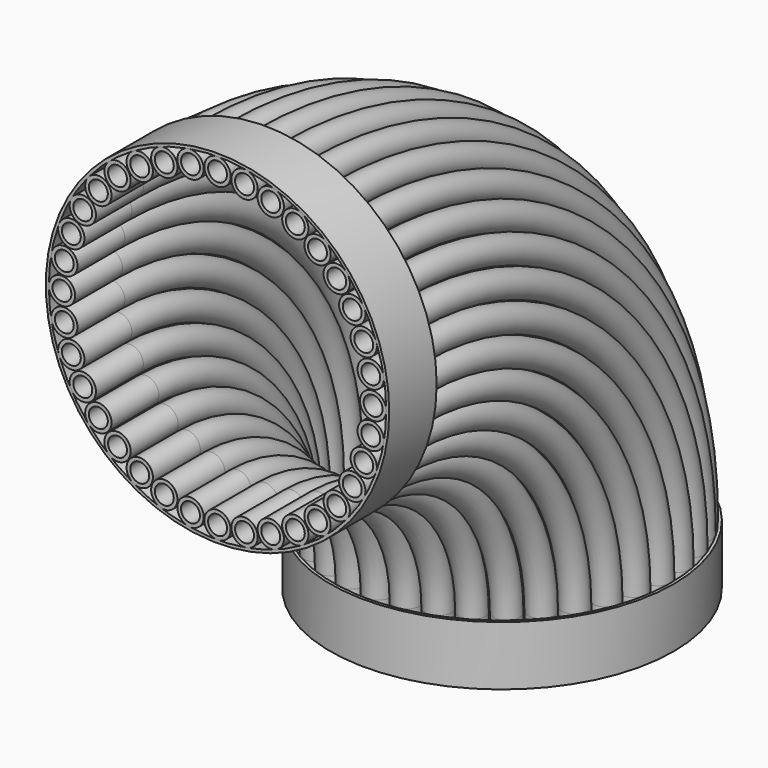
from build123d import *

# Parameters (mm, degrees)
F0_R     = 44.45
F0_R_2   = 31.95
F3_R     = 579.45
F3_R_2   = 569.45
F4_DEPTH = 200
F6_R     = 579.45
F6_R_2   = 569.45
F7_DEPTH = 200


with BuildPart() as f2:
    # F2: sweep along a path in F1
    with BuildLine(Plane.YZ) as f2_path:
        Line((0, 0), (200, 0))
        ThreePointArc((200, 0), (907.1067811865, -292.8932188135), (1200, -1000))
        Line((1200, -1000), (1200, -1200))
    # F0 (on Front) → F2 (sweep)
    with BuildSketch(Plane.XZ):
        with Locations((0, 525)):
            Circle(F0_R)
        with Locations((0, 525)):
            Circle(F0_R_2, mode=Mode.SUBTRACT)
        with Locations((-91.1652932751, 517.0240703314)):
            Circle(F0_R)
        with Locations((-91.1652932751, 517.0240703314)):
            Circle(F0_R_2, mode=Mode.SUBTRACT)
        with Locations((-179.560575246, 493.3386259126)):
            Circle(F0_R)
        with Locations((-179.560575246, 493.3386259126)):
            Circle(F0_R_2, mode=Mode.SUBTRACT)
        with Locations((-262.5, 454.6633369868)):
            Circle(F0_R)
        with Locations((-262.5, 454.6633369868)):
            Circle(F0_R_2, mode=Mode.SUBTRACT)
        with Locations((-337.4634950854, 402.1733326375)):
            Circle(F0_R)
        with Locations((-337.4634950854, 402.1733326375)):
            Circle(F0_R_2, mode=Mode.SUBTRACT)
        with Locations((-402.1733326375, 337.4634950854)):
            Circle(F0_R)
        with Locations((-402.1733326375, 337.4634950854)):
            Circle(F0_R_2, mode=Mode.SUBTRACT)
        with Locations((-454.6633369868, 262.5)):
            Circle(F0_R)
        with Locations((-454.6633369868, 262.5)):
            Circle(F0_R_2, mode=Mode.SUBTRACT)
        with Locations((-493.3386259126, 179.560575246)):
            Circle(F0_R)
        with Locations((-493.3386259126, 179.560575246)):
            Circle(F0_R_2, mode=Mode.SUBTRACT)
        with Locations((-517.0240703314, 91.1652932751)):
            Circle(F0_R)
        with Locations((-517.0240703314, 91.1652932751)):
            Circle(F0_R_2, mode=Mode.SUBTRACT)
        with Locations((-525, 0)):
            Circle(F0_R)
        with Locations((-525, 0)):
            Circle(F0_R_2, mode=Mode.SUBTRACT)
        with Locations((-517.0240703314, -91.1652932751)):
            Circle(F0_R)
        with Locations((-517.0240703314, -91.1652932751)):
            Circle(F0_R_2, mode=Mode.SUBTRACT)
        with Locations((-493.3386259126, -179.560575246)):
            Circle(F0_R)
        with Locations((-493.3386259126, -179.560575246)):
            Circle(F0_R_2, mode=Mode.SUBTRACT)
        with Locations((-454.6633369868, -262.5)):
            Circle(F0_R)
        with Locations((-454.6633369868, -262.5)):
            Circle(F0_R_2, mode=Mode.SUBTRACT)
        with Locations((-402.1733326375, -337.4634950854)):
            Circle(F0_R)
        with Locations((-402.1733326375, -337.4634950854)):
            Circle(F0_R_2, mode=Mode.SUBTRACT)
        with Locations((-337.4634950854, -402.1733326375)):
            Circle(F0_R)
        with Locations((-337.4634950854, -402.1733326375)):
            Circle(F0_R_2, mode=Mode.SUBTRACT)
        with Locations((-262.5, -454.6633369868)):
            Circle(F0_R)
        with Locations((-262.5, -454.6633369868)):
            Circle(F0_R_2, mode=Mode.SUBTRACT)
        with Locations((-179.560575246, -493.3386259126)):
            Circle(F0_R)
        with Locations((-179.560575246, -493.3386259126)):
            Circle(F0_R_2, mode=Mode.SUBTRACT)
        with Locations((-91.1652932751, -517.0240703314)):
            Circle(F0_R)
        with Locations((-91.1652932751, -517.0240703314)):
            Circle(F0_R_2, mode=Mode.SUBTRACT)
        with Locations((0, -525)):
            Circle(F0_R)
        with Locations((0, -525)):
            Circle(F0_R_2, mode=Mode.SUBTRACT)
        with Locations((91.1652932751, -517.0240703314)):
            Circle(F0_R)
        with Locations((91.1652932751, -517.0240703314)):
            Circle(F0_R_2, mode=Mode.SUBTRACT)
        with Locations((179.560575246, -493.3386259126)):
            Circle(F0_R)
        with Locations((179.560575246, -493.3386259126)):
            Circle(F0_R_2, mode=Mode.SUBTRACT)
        with Locations((262.5, -454.6633369868)):
            Circle(F0_R)
        with Locations((262.5, -454.6633369868)):
            Circle(F0_R_2, mode=Mode.SUBTRACT)
        with Locations((337.4634950854, -402.1733326375)):
            Circle(F0_R)
        with Locations((337.4634950854, -402.1733326375)):
            Circle(F0_R_2, mode=Mode.SUBTRACT)
        with Locations((402.1733326375, -337.4634950854)):
            Circle(F0_R)
        with Locations((402.1733326375, -337.4634950854)):
            Circle(F0_R_2, mode=Mode.SUBTRACT)
        with Locations((454.6633369868, -262.5)):
            Circle(F0_R)
        with Locations((454.6633369868, -262.5)):
            Circle(F0_R_2, mode=Mode.SUBTRACT)
        with Locations((493.3386259126, -179.560575246)):
            Circle(F0_R)
        with Locations((493.3386259126, -179.560575246)):
            Circle(F0_R_2, mode=Mode.SUBTRACT)
        with Locations((517.0240703314, -91.1652932751)):
            Circle(F0_R)
        with Locations((517.0240703314, -91.1652932751)):
            Circle(F0_R_2, mode=Mode.SUBTRACT)
        with Locations((525, 0)):
            Circle(F0_R)
        with Locations((525, 0)):
            Circle(F0_R_2, mode=Mode.SUBTRACT)
        with Locations((517.0240703314, 91.1652932751)):
            Circle(F0_R)
        with Locations((517.0240703314, 91.1652932751)):
            Circle(F0_R_2, mode=Mode.SUBTRACT)
        with Locations((493.3386259126, 179.560575246)):
            Circle(F0_R)
        with Locations((493.3386259126, 179.560575246)):
            Circle(F0_R_2, mode=Mode.SUBTRACT)
        with Locations((454.6633369868, 262.5)):
            Circle(F0_R)
        with Locations((454.6633369868, 262.5)):
            Circle(F0_R_2, mode=Mode.SUBTRACT)
        with Locations((402.1733326375, 337.4634950854)):
            Circle(F0_R)
        with Locations((402.1733326375, 337.4634950854)):
            Circle(F0_R_2, mode=Mode.SUBTRACT)
        with Locations((337.4634950854, 402.1733326375)):
            Circle(F0_R)
        with Locations((337.4634950854, 402.1733326375)):
            Circle(F0_R_2, mode=Mode.SUBTRACT)
        with Locations((262.5, 454.6633369868)):
            Circle(F0_R)
        with Locations((262.5, 454.6633369868)):
            Circle(F0_R_2, mode=Mode.SUBTRACT)
        with Locations((179.560575246, 493.3386259126)):
            Circle(F0_R)
        with Locations((179.560575246, 493.3386259126)):
            Circle(F0_R_2, mode=Mode.SUBTRACT)
        with Locations((91.1652932751, 517.0240703314)):
            Circle(F0_R)
        with Locations((91.1652932751, 517.0240703314)):
            Circle(F0_R_2, mode=Mode.SUBTRACT)
    sweep(path=f2_path.line)


with BuildPart() as f4:
    # F3 (on Front) → F4 (new body)
    with BuildSketch(Plane.XZ):
        Circle(F3_R)
        Circle(F3_R_2, mode=Mode.SUBTRACT)
    extrude(amount=-F4_DEPTH)


with BuildPart() as f7:
    # F6 (on line) → F7 (new body)
    with BuildSketch(Plane(origin=(0, 0, -1200), x_dir=(1, 0, 0), z_dir=(0, 0, -1))):
        with Locations((0, -1200)):
            Circle(F6_R)
        with Locations((0, -1200)):
            Circle(F6_R_2, mode=Mode.SUBTRACT)
    extrude(amount=-F7_DEPTH)


solid = Compound([f2.part, f4.part, f7.part])
